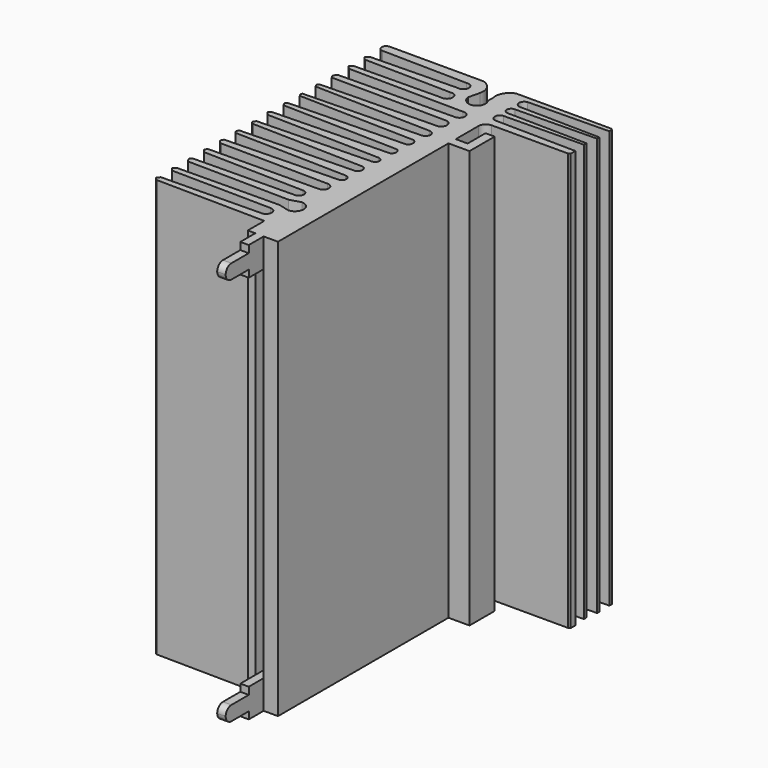
from build123d import *

# Parameters (mm, degrees)
F1_DEPTH = 29
F2_START = 25
F2_DEPTH = 4
F3_START = -25
F3_DEPTH = 4
F4_START = 26
F0_W     = 1.172746277
F0_H     = 3.0541475862
F0_H_2   = 0.957692816
F4_DEPTH = 2
F5_START = -26
F5_DEPTH = 2
F6_R     = 0.99999


# Not quite as in the source:
# - a fillet or chamfer is up to 0.001 mm smaller than in the source, because OpenCascade refuses the exact size


with BuildPart() as f1:
    # F0 (on Top) → F1 (new body, symmetric)
    with BuildSketch(Plane.XY):
        with BuildLine():
            Line((-4.0699890815, 24.2982581258), (-17.1110220253, 24.2982581258))
            ThreePointArc((-17.1110220253, 24.2982581258), (-17.7348526195, 23.6744275317), (-17.1110220253, 23.0505969375))
            Line((-17.1110220253, 23.0505969375), (-5.313185975, 22.8393822908))
            ThreePointArc((-5.313185975, 22.8393822908), (-4.3551853687, 22.085041739), (-5.313185975, 21.3307011873))
            Line((-5.313185975, 21.3307011873), (-17.3267684877, 21.0792534053))
            Line((-17.3267684877, 21.0792534053), (-17.7458468825, 20.7020826638))
            Line((-17.7458468825, 20.7020826638), (-17.3267684877, 20.2364402329))
            Line((-17.3267684877, 20.2364402329), (-5.313185975, 20.0213631141))
            ThreePointArc((-5.313185975, 20.0213631141), (-4.319986106, 19.2441805029), (-5.313185975, 18.4669978917))
            Line((-5.313185975, 18.4669978917), (-17.3407383263, 18.3133352548))
            Line((-17.3407383263, 18.3133352548), (-17.7458468825, 17.9431512952))
            Line((-17.7458468825, 17.9431512952), (-17.3407383263, 17.4823310226))
            Line((-17.3407383263, 17.4823310226), (-1.3890911359, 17.3372328281))
            ThreePointArc((-1.3890911359, 17.3372328281), (-0.492008259, 16.5730640292), (-1.3890911359, 15.8088952303))
            Line((-1.3890911359, 15.8088952303), (-17.3541552482, 15.6049273923))
            Line((-17.3541552482, 15.6049273923), (-17.7356619388, 15.1443993673))
            Line((-17.7356619388, 15.1443993673), (-17.5030883402, 14.7124780342))
            Line((-17.5030883402, 14.7124780342), (-1.3890911359, 14.5659030835))
            ThreePointArc((-1.3890911359, 14.5659030835), (-0.7437511811, 13.7670414267), (-1.3890911359, 12.9681797698))
            Line((-1.3890911359, 12.9681797698), (-17.4349947409, 12.6323343327))
            Line((-17.4349947409, 12.6323343327), (-17.7414808422, 12.3967602849))
            Line((-17.7414808422, 12.3967602849), (-17.5598803908, 11.9637120515))
            Line((-17.5598803908, 11.9637120515), (-1.3890911359, 11.5619925782))
            ThreePointArc((-1.3890911359, 11.5619925782), (-0.7146102661, 10.8705479652), (-1.3890911359, 10.1791033521))
            Line((-1.3890911359, 10.1791033521), (-17.4349947409, 9.7804863246))
            Line((-17.4349947409, 9.7804863246), (-17.57148467, 9.7804863246))
            Line((-17.57148467, 9.7804863246), (-17.7426468581, 9.5952115953))
            Line((-17.7426468581, 9.5952115953), (-17.5253339112, 9.1899503022))
            Line((-17.5253339112, 9.1899503022), (-1.3890911359, 8.7890890427))
            ThreePointArc((-1.3890911359, 8.7890890427), (-0.9606665076, 8.1417476758), (-1.3890911359, 7.494406309))
            Line((-1.3890911359, 7.494406309), (-17.5261050463, 7.0715243928))
            Line((-17.5261050463, 7.0715243928), (-17.7610386163, 6.8365903571))
            Line((-17.7610386163, 6.8365903571), (-17.5261050463, 6.3615223657))
            Line((-17.5261050463, 6.3615223657), (-1.3890911359, 5.9555862099))
            ThreePointArc((-1.3890911359, 5.9555862099), (-1.0583889027, 5.3565036505), (-1.3890911359, 4.7574210912))
            Line((-1.3890911359, 4.7574210912), (-17.4686410496, 4.3360450599))
            Line((-17.4686410496, 4.3360450599), (-17.8654273587, 3.982137423))
            Line((-17.8654273587, 3.982137423), (-17.4686410496, 3.5372773558))
            Line((-17.4686410496, 3.5372773558), (-1.7663730541, 3.1859290281))
            ThreePointArc((-1.7663730541, 3.1859290281), (-1.2007925503, 2.6075517307), (-1.7663730541, 2.0291744333))
            Line((-1.7663730541, 2.0291744333), (-17.4686410496, 1.6176853427))
            Line((-17.4686410496, 1.6176853427), (-17.7483521402, 1.1909720488))
            Line((-17.7483521402, 1.1909720488), (-17.4686410496, 0.8753370494))
            Line((-17.4686410496, 0.8753370494), (-1.7663730541, 0.4803371849))
            ThreePointArc((-1.7663730541, 0.4803371849), (-1.3259179646, -0.1754465338), (-1.7663730541, -0.8312302525))
            Line((-1.7663730541, -0.8312302525), (-17.5491847508, -1.244830048))
            ThreePointArc((-17.5491847508, -1.244830048), (-17.7110050083, -1.6010632209), (-17.5491847508, -1.9572963938))
            Line((-17.5491847508, -1.9572963938), (-1.9620249514, -2.3128963076))
            ThreePointArc((-1.9620249514, -2.3128963076), (-1.3537602225, -2.9351960402), (-1.9620249514, -3.5574957728))
            Line((-1.9620249514, -3.5574957728), (-17.5113877616, -3.9649778744))
            Line((-17.5113877616, -3.9649778744), (-17.7269522101, -4.4069844298))
            Line((-17.7269522101, -4.4069844298), (-17.312085256, -4.8613618128))
            Line((-17.312085256, -4.8613618128), (-2.2583589889, -5.0391620025))
            ThreePointArc((-2.2583589889, -5.0391620025), (-1.4871772278, -5.8195060119), (-2.2583589889, -6.5998500213))
            Line((-2.2583589889, -6.5998500213), (-17.5293660294, -6.7802165233))
            Line((-17.5293660294, -6.7802165233), (-17.7314169705, -7.1995011531))
            Line((-17.7314169705, -7.1995011531), (-17.3472613096, -7.6185795479))
            Line((-17.3472613096, -7.6185795479), (-3.3617539701, -7.9376399327))
            ThreePointArc((-3.3617539701, -7.9376399327), (-2.6814550827, -8.6336359286), (-3.3617539701, -9.3296319246))
            Line((-3.3617539701, -9.3296319246), (-17.4733772874, -9.5469430089))
            Line((-17.4733772874, -9.5469430089), (-17.710454762, -9.9222976714))
            Line((-17.710454762, -9.9222976714), (-17.335081473, -10.4161864147))
            Line((-17.335081473, -10.4161864147), (-3.228909336, -10.6137422845))
            Line((-3.228909336, -10.6137422845), (-1.7076556105, -10.1791201159))
            ThreePointArc((-1.7076556105, -10.1791201159), (-0.5341015375, -11.3842086866), (-1.7076556105, -12.5892972574))
            Line((-1.7076556105, -12.5892972574), (-3.189396346, -12.1941864491))
            Line((-3.189396346, -12.1941864491), (-17.2815993428, -12.3514840379))
            Line((-17.2815993428, -12.3514840379), (-17.7286379039, -12.7565935254))
            Line((-17.7286379039, -12.7565935254), (-17.3566557611, -13.1670760419))
            Line((-17.3566557611, -13.1670760419), (-3.5123708679, -13.3609642008))
            ThreePointArc((-3.5123708679, -13.3609642008), (-2.7387752862, -14.1454697919), (-3.5123708679, -14.929975383))
            Line((-3.5123708679, -14.929975383), (-17.3472613096, -15.1430249362))
            Line((-17.3472613096, -15.1430249362), (-17.6943112165, -15.5275696889))
            Line((-17.6943112165, -15.5275696889), (-17.3472613096, -15.9387048334))
            Line((-17.3472613096, -15.9387048334), (-2.1711152967, -16.1512456061))
            Line((-2.1711152967, -16.1512456061), (-2.1711152967, -19.0259180963))
            Line((-2.1711152967, -19.0259180963), (-1.1235726997, -19.0259180963))
            Line((-1.1235726997, -19.0259180963), (-1.1235726997, -15.1430249362))
            Line((-1.1235726997, -15.1430249362), (0.0491735773, -15.1430249362))
            Line((0.0491735773, -15.1430249362), (0.0491735773, -19.047325477))
            Line((0.0491735773, -19.047325477), (2.0417859778, -19.047325477))
            Line((2.0417859778, -19.047325477), (2.0417859778, 10.5479126796))
            Line((2.0417859778, 10.5479126796), (4.9630478024, 10.5479126796))
            Line((4.9630478024, 10.5479126796), (4.9630478024, 14.9210141972))
            Line((4.9630478024, 14.9210141972), (3.692939326, 14.901455239))
            Line((3.692939326, 14.901455239), (3.692939326, 11.8128489703))
            Line((3.692939326, 11.8128489703), (2.0417859778, 11.8128489703))
            Line((2.0417859778, 11.8128489703), (2.0417859778, 15.7654304057))
            ThreePointArc((2.0417859778, 15.7654304057), (2.3413387619, 16.4847297298), (3.0629034154, 16.7787838727))
            Line((3.0629034154, 16.7787838727), (13.6287314817, 16.7787838727))
            Line((13.6287314817, 16.7787838727), (13.9106530696, 16.9266853482))
            Line((13.9106530696, 16.9266853482), (13.9106530696, 17.7426013646))
            Line((13.9106530696, 17.7426013646), (2.7096215636, 17.9149005562))
            ThreePointArc((2.7096215636, 17.9149005562), (2.027143744, 18.6079572886), (2.7096215636, 19.301014021))
            Line((2.7096215636, 19.301014021), (13.7074142694, 19.4701869041))
            Line((13.7074142694, 19.4701869041), (13.7007343839, 19.9044408738))
            Line((13.7007343839, 19.9044408738), (2.7096215636, 20.0889185071))
            ThreePointArc((2.7096215636, 20.0889185071), (2.0410304994, 20.6815851852), (2.7096215636, 21.2742518634))
            Line((2.7096215636, 21.2742518634), (13.9556201175, 21.4712414891))
            Line((13.9556201175, 21.4712414891), (13.9486206756, 21.8708346796))
            Line((13.9486206756, 21.8708346796), (2.7096215636, 22.0614876598))
            ThreePointArc((2.7096215636, 22.0614876598), (2.0808096295, 22.7669365704), (2.7096215636, 23.472385481))
            Line((2.7096215636, 23.472385481), (13.9058372006, 23.6605741084))
            Line((13.9058372006, 23.6605741084), (13.8986392592, 24.088813075))
            Line((13.8986392592, 24.088813075), (13.6943962425, 24.271402508))
            Line((13.6943962425, 24.271402508), (0.4630363837, 24.271402508))
            ThreePointArc((0.4630363837, 24.271402508), (-0.6487056649, 23.3676230344), (-0.8640453452, 21.9511426985))
            Line((-0.8640453452, 21.9511426985), (-0.8640453452, 21.0152007639))
            ThreePointArc((-0.8640453452, 21.0152007639), (-0.7734316844, 19.7347502036), (-1.897772192, 19.1153772175))
            ThreePointArc((-1.897772192, 19.1153772175), (-2.6726628699, 19.513906378), (-3.0711919535, 20.2887970954))
            Line((-3.0711919535, 20.2887970954), (-2.680051839, 21.9092350453))
            ThreePointArc((-2.680051839, 21.9092350453), (-2.8952979424, 23.3828498722), (-4.0699890815, 24.2982581258))
        make_face()
    extrude(amount=F1_DEPTH, both=True)

    # F0 (on Top) → F2 (join)
    with BuildSketch(Plane.XY.offset(F2_START)):
        Polygon((0.0491735773, -21.6273944825), (0.0491735773, -19.047325477), (0.0491735773, -15.1430249362), (-1.1235726997, -15.1430249362), (-1.1235726997, -19.0259180963), (-1.1235726997, -21.6273944825), align=None)
    extrude(amount=F2_DEPTH)

    # F0 (on Top) → F3 (join)
    with BuildSketch(Plane.XY.offset(F3_START)):
        Polygon((0.0491735773, -21.6273944825), (0.0491735773, -19.047325477), (0.0491735773, -15.1430249362), (-1.1235726997, -15.1430249362), (-1.1235726997, -19.0259180963), (-1.1235726997, -21.6273944825), align=None)
    extrude(amount=-F3_DEPTH)

    # F0 (on Top) → F4 (join)
    with BuildSketch(Plane.XY.offset(F4_START)):
        with Locations((-0.5371995612, -23.1544682756)):
            Rectangle(F0_W, F0_H)
        with Locations((-0.5371995612, -25.1603884767)):
            Rectangle(F0_W, F0_H_2)
    extrude(amount=F4_DEPTH)

    # F0 (on Top) → F5 (join)
    with BuildSketch(Plane.XY.offset(F5_START)):
        with Locations((-0.5371995612, -23.1544682756)):
            Rectangle(F0_W, F0_H)
        with Locations((-0.5371995612, -25.1603884767)):
            Rectangle(F0_W, F0_H_2)
    extrude(amount=-F5_DEPTH)

    # F6 (radius 1 in the source; OpenCascade refuses exactly that, so slightly less here)
    f6_edges = [f1.edges().sort_by_distance(p)[0] for p in [
        (-0.5372, -25.639235, 28),
        (-0.5372, -25.639235, 26),
        (-0.5372, -25.639235, -26),
        (-0.5372, -25.639235, -28),
    ]]
    fillet(f6_edges, radius=F6_R)


solid = f1.part
